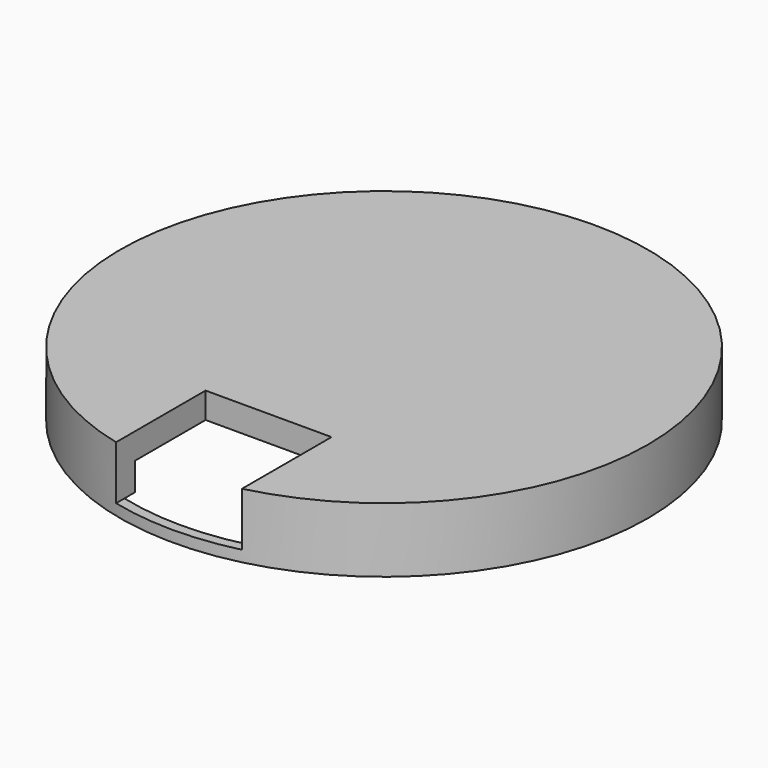
from build123d import *

# Parameters (mm, degrees)
F0_R     = 13.5
F0_W     = 6
F0_H     = 4.25
F1_DEPTH = 1.2
F2_DEPTH = 4.2
F3_R     = 14.25
F3_R_2   = 13.7
F3_R_3   = 13.5
F4_DEPTH = 2.9
F5_DEPTH = 0.6
F3_W     = 6
F3_H     = 4.25
F6_DEPTH = 1.5
F7_W     = 6.8
F7_H     = 3
F8_DEPTH = 8


with BuildPart() as f1:
    # F0 (on Top) → F1 (new body)
    with BuildSketch(Plane.XY):
        Circle(F0_R)
        with Locations((0, -10.295)):
            Rectangle(F0_W, F0_H, mode=Mode.SUBTRACT)
        with Locations((0, -10.295)):
            Rectangle(F0_W, F0_H)
    extrude(amount=F1_DEPTH)

    # F0 (on Top) → F2 (join)
    with BuildSketch(Plane.XY):
        with Locations((0, -10.295)):
            Rectangle(F0_W, F0_H)
    extrude(amount=F2_DEPTH)


with BuildPart() as f4:
    # F3 (on face) → F4 (new body)
    with BuildSketch(Plane.XY.offset(1.2)):
        Circle(F3_R)
        Circle(F3_R_2, mode=Mode.SUBTRACT)
        Circle(F3_R_2)
        Circle(F3_R_3, mode=Mode.SUBTRACT)
        Circle(F3_R_3)
        with BuildLine():
            Line((3.4, -12.5475097131), (3.4, -12.795))
            Line((3.4, -12.795), (2.2995597405, -12.795))
            ThreePointArc((2.2995597405, -12.795), (0, -13), (-2.2995597405, -12.795))
            Line((-2.2995597405, -12.795), (-3.4, -12.795))
            Line((-3.4, -12.795), (-3.4, -12.5475097131))
            ThreePointArc((-3.4, -12.5475097131), (-7.8993670633, 10.3247275993), (13, 0))
            ThreePointArc((13, 0), (10.3247275993, -7.8993670633), (3.4, -12.5475097131))
        make_face(mode=Mode.SUBTRACT)
        with BuildLine():
            Line((3.4, -7.795), (3.4, -12.5475097131))
            ThreePointArc((3.4, -12.5475097131), (10.3247275993, -7.8993670633), (13, 0))
            ThreePointArc((13, 0), (-7.8993670633, 10.3247275993), (-3.4, -12.5475097131))
            Line((-3.4, -12.5475097131), (-3.4, -7.795))
            Line((-3.4, -7.795), (3.4, -7.795))
        make_face()
        with BuildLine():
            ThreePointArc((-2.2995597405, -12.795), (0, -13), (2.2995597405, -12.795))
            Line((2.2995597405, -12.795), (-2.2995597405, -12.795))
        make_face()
    extrude(amount=F4_DEPTH)

    # F3 (on face) → F5 (join)
    with BuildSketch(Plane.XY.offset(1.2)):
        Circle(F3_R)
        Circle(F3_R_2, mode=Mode.SUBTRACT)
    extrude(amount=-F5_DEPTH)

    # F3 (on face) → F6 (cut)
    with BuildSketch(Plane.XY.offset(1.2)):
        with BuildLine():
            Line((3.4, -7.795), (3.4, -12.5475097131))
            ThreePointArc((3.4, -12.5475097131), (10.3247275993, -7.8993670633), (13, 0))
            ThreePointArc((13, 0), (-7.8993670633, 10.3247275993), (-3.4, -12.5475097131))
            Line((-3.4, -12.5475097131), (-3.4, -7.795))
            Line((-3.4, -7.795), (3.4, -7.795))
        make_face()
        with BuildLine():
            Line((-2.2995597405, -12.795), (2.2995597405, -12.795))
            ThreePointArc((2.2995597405, -12.795), (2.8524652793, -12.6831952532), (3.4, -12.5475097131))
            Line((3.4, -12.5475097131), (3.4, -7.795))
            Line((3.4, -7.795), (-3.4, -7.795))
            Line((-3.4, -7.795), (-3.4, -12.5475097131))
            ThreePointArc((-3.4, -12.5475097131), (-2.8524652793, -12.6831952532), (-2.2995597405, -12.795))
        make_face()
        with Locations((0, -10.295)):
            Rectangle(F3_W, F3_H, mode=Mode.SUBTRACT)
        with BuildLine():
            ThreePointArc((-2.2995597405, -12.795), (0, -13), (2.2995597405, -12.795))
            Line((2.2995597405, -12.795), (-2.2995597405, -12.795))
        make_face()
    extrude(amount=F6_DEPTH, mode=Mode.SUBTRACT)

    # F7 (on face) → F8 (cut)
    with BuildSketch(Plane.XZ.offset(12.42)):
        with Locations((0, 2.7)):
            Rectangle(F7_W, F7_H)
    extrude(amount=F8_DEPTH, mode=Mode.SUBTRACT)


solid = f4.part
